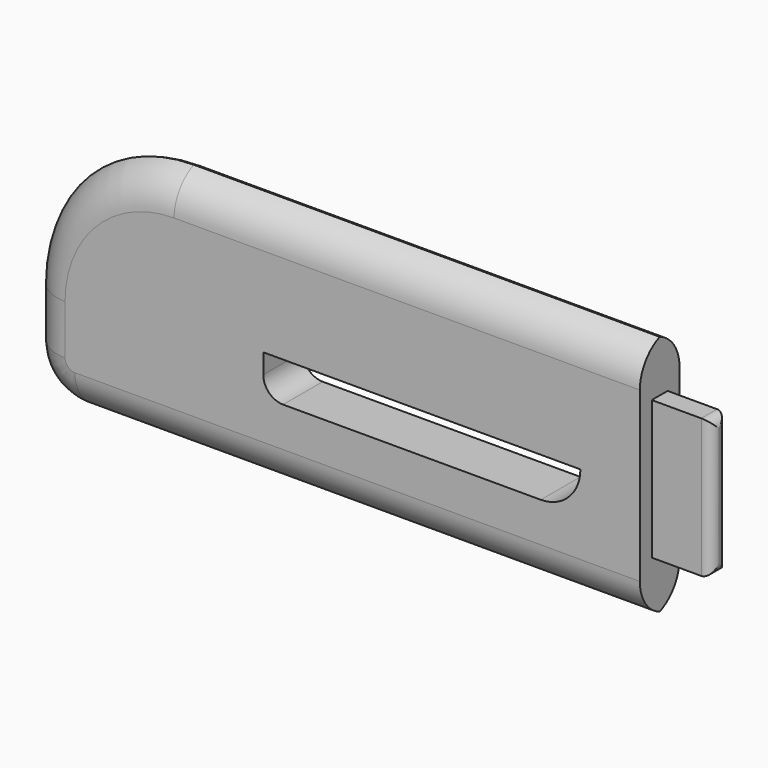
from build123d import *

# Parameters (mm, degrees)
F0_W         = 40.64
F0_H         = 5.08
F1_DEPTH     = 6.35
F3_DEPTH     = 7.62
F4_R         = 1.26999
F5_T1_DEPTH  = 6.35
F5_T3_DEPTH  = 85.09
F5_T5_DEPTH  = 72.39
F5_T8_ANGLE  = 90
F5_T10_ANGLE = 90
F5_T12_ANGLE = 90
F5_T14_ANGLE = 90
F6_R         = 5.07999
F7_R         = 2.54


# Not quite as in the source:
# - a fillet or chamfer that OpenCascade refuses, or shapes differently, is made with other operations: its cross-section is extruded or revolved along the edge and cut away or added
# - a fillet or chamfer is up to 0.001 mm smaller than in the source, because OpenCascade refuses the exact size


with BuildPart() as f1:
    # F0 (on Front) → F1 (new body)
    with BuildSketch(Plane.XZ):
        with BuildLine():
            ThreePointArc((-31.75, 19.05), (-45.2203841816, 13.4703841816), (-50.8, 0))
            Line((-50.8, 0), (-50.8, -6.35))
            ThreePointArc((-50.8, -6.35), (-48.9401280605, -10.8401280605), (-44.45, -12.7))
            Line((-44.45, -12.7), (27.94, -12.7))
            Line((27.94, -12.7), (27.94, 19.05))
            Line((27.94, 19.05), (20.32, 19.05))
            Line((20.32, 19.05), (-31.75, 19.05))
        make_face()
        Rectangle(F0_W, F0_H, mode=Mode.SUBTRACT)
    extrude(amount=F1_DEPTH)

    # F2 (on face) → F3 (join)
    with BuildSketch(Plane.YZ.offset(27.94)):
        Polygon((-4.445, -5.715), (-3.175, -5.715), (-1.905, -5.715), (-1.905, 12.065), (-4.445, 12.065), align=None)
    extrude(amount=F3_DEPTH)

    # F4 (radius 1.27 in the source; OpenCascade refuses exactly that, so slightly less here)
    f4_edges = [f1.edges().sort_by_distance(p)[0] for p in [
        (35.56, -4.445, 3.175),
        (35.56, -3.175, 12.065),
        (35.56, -1.905, 3.175),
        (35.56, -3.175, -5.715),
    ]]
    fillet(f4_edges, radius=F4_R)

    # F5: fillet of radius 5.08 on 2 edges, made by hand

    # F5_s2 → F5_t1 (cut)
    with BuildSketch(Plane.XY.offset(-6.35)):
        with BuildLine():
            ThreePointArc((-45.72, 0), (-49.3121024484, -1.4878975516), (-50.8, -5.08))
            Line((-50.8, -5.08), (-50.8, 0))
            Line((-50.8, 0), (-45.72, 0))
        make_face()
        with BuildLine():
            ThreePointArc((-45.72, -6.35), (-49.3121024484, -4.8621024484), (-50.8, -1.27))
            Line((-50.8, -1.27), (-50.8, -6.35))
            Line((-50.8, -6.35), (-45.72, -6.35))
        make_face()
    extrude(amount=F5_T1_DEPTH, mode=Mode.SUBTRACT)

    # F5_s4 → F5_t3 (cut)
    with BuildSketch(Plane.YZ.offset(-44.45)):
        with BuildLine():
            ThreePointArc((-5.08, -12.7), (-1.4878975516, -11.2121024484), (0, -7.62))
            Line((0, -7.62), (0, -12.7))
            Line((0, -12.7), (-5.08, -12.7))
        make_face()
        with BuildLine():
            ThreePointArc((-1.27, -12.7), (-4.8621024484, -11.2121024484), (-6.35, -7.62))
            Line((-6.35, -7.62), (-6.35, -12.7))
            Line((-6.35, -12.7), (-1.27, -12.7))
        make_face()
    extrude(amount=F5_T3_DEPTH, mode=Mode.SUBTRACT)

    # F5_s6 → F5_t5 (cut)
    with BuildSketch(Plane.YZ.offset(-31.75)):
        with BuildLine():
            ThreePointArc((0, 13.97), (-1.4878975516, 17.5621024484), (-5.08, 19.05))
            Line((-5.08, 19.05), (0, 19.05))
            Line((0, 19.05), (0, 13.97))
        make_face()
        with BuildLine():
            ThreePointArc((-6.35, 13.97), (-4.8621024484, 17.5621024484), (-1.27, 19.05))
            Line((-1.27, 19.05), (-6.35, 19.05))
            Line((-6.35, 19.05), (-6.35, 13.97))
        make_face()
    extrude(amount=F5_T5_DEPTH, mode=Mode.SUBTRACT)

    # F5_s7 → F5_t8 (revolve, cut)
    with BuildSketch(Plane.XY.offset(-6.35)):
        with BuildLine():
            ThreePointArc((-45.72, -6.35), (-49.3121024484, -4.8621024484), (-50.8, -1.27))
            Line((-50.8, -1.27), (-50.8, -6.35))
            Line((-50.8, -6.35), (-45.72, -6.35))
        make_face()
    revolve(axis=Axis((-44.45, -6.35, -6.35), (0, -1, 0)), revolution_arc=F5_T8_ANGLE, mode=Mode.SUBTRACT)

    # F5_s9 → F5_t10 (revolve, cut)
    with BuildSketch(Plane.YZ.offset(-31.75)):
        with BuildLine():
            ThreePointArc((0, 13.97), (-1.4878975516, 17.5621024484), (-5.08, 19.05))
            Line((-5.08, 19.05), (0, 19.05))
            Line((0, 19.05), (0, 13.97))
        make_face()
    revolve(axis=Axis((-31.75, 0, 0), (0, -1, 0)), revolution_arc=F5_T10_ANGLE, mode=Mode.SUBTRACT)

    # F5_s11 → F5_t12 (revolve, cut)
    with BuildSketch(Plane.XY.offset(-6.35)):
        with BuildLine():
            ThreePointArc((-45.72, 0), (-49.3121024484, -1.4878975516), (-50.8, -5.08))
            Line((-50.8, -5.08), (-50.8, 0))
            Line((-50.8, 0), (-45.72, 0))
        make_face()
    revolve(axis=Axis((-44.45, 0, -6.35), (0, -1, 0)), revolution_arc=F5_T12_ANGLE, mode=Mode.SUBTRACT)

    # F5_s13 → F5_t14 (revolve, cut)
    with BuildSketch(Plane.YZ.offset(-31.75)):
        with BuildLine():
            ThreePointArc((-6.35, 13.97), (-4.8621024484, 17.5621024484), (-1.27, 19.05))
            Line((-1.27, 19.05), (-6.35, 19.05))
            Line((-6.35, 19.05), (-6.35, 13.97))
        make_face()
    revolve(axis=Axis((-31.75, -6.35, 0), (0, -1, 0)), revolution_arc=F5_T14_ANGLE, mode=Mode.SUBTRACT)

    # F6 (radius 5.08 in the source; OpenCascade refuses exactly that, so slightly less here)
    f6_edges = [f1.edges().sort_by_distance(p)[0] for p in [
        (20.32, -3.175, -2.54),
    ]]
    fillet(f6_edges, radius=F6_R)

    # F7
    f7_edges = [f1.edges().sort_by_distance(p)[0] for p in [
        (-20.32, -3.175, -2.54),
    ]]
    fillet(f7_edges, radius=F7_R)


solid = f1.part
